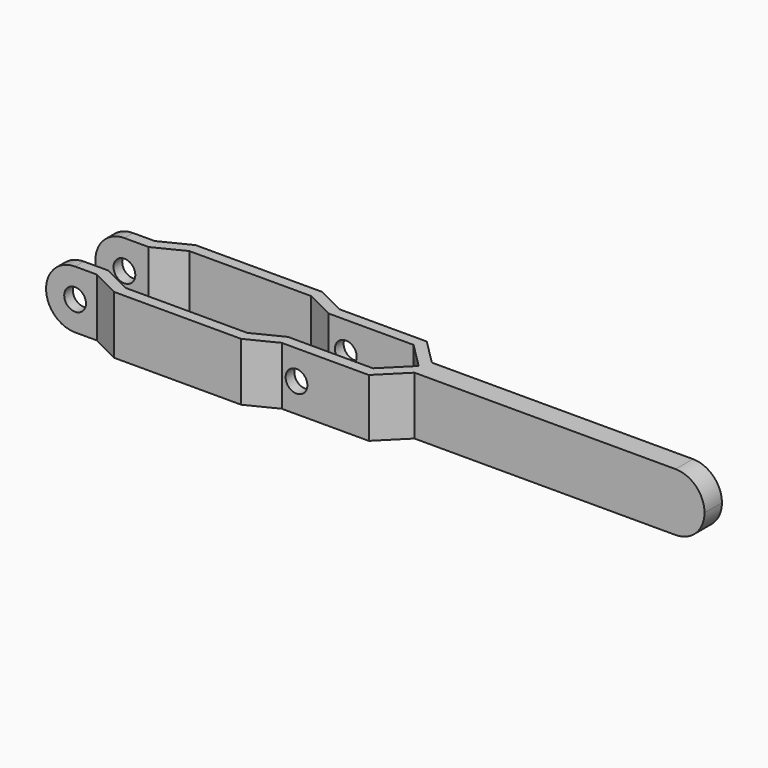
from build123d import *

# Parameters (mm, degrees)
F1_DEPTH = 16
F3_W     = 3
F3_H     = 16
F5_DEPTH = 8
F4_W     = 6
F4_H     = 16
F6_DEPTH = 8
F7_D     = 6
F8_R     = 7.99999


# Not quite as in the source:
# - a fillet or chamfer is up to 0.001 mm smaller than in the source, because OpenCascade refuses the exact size


with BuildPart() as f1:
    # F0 (on Top) → F1 (new body)
    with BuildSketch(Plane.XY):
        Polygon((-80.7573593129, 10), (-86.7573593129, 10), (-86.7573593129, 7), (-80.0491553804, 7), (-72.0491553804, 11), (-38.4655632454, 11), (-30.4655632454, 7), (-7, 7), (0, 0), (-7, -7), (-30.4655632454, -7), (-38.4655632454, -11), (-72.0491553804, -11), (-80.0491553804, -7), (-86.7573593129, -7), (-86.7573593129, -10), (-80.7573593129, -10), (-72.7573593129, -14), (-37.7573593129, -14), (-29.7573593129, -10), (-5.7573593129, -10), (1.2426406871, -3), (73.2426406871, -3), (73.2426406871, 3), (1.2426406871, 3), (-5.7573593129, 10), (-29.7573593129, 10), (-37.7573593129, 14), (-72.7573593129, 14), align=None)
    extrude(amount=F1_DEPTH)

    # F3 (on face) → F5 (join)
    with BuildSketch(Plane(origin=(-86.7573593129, 0, 0), x_dir=(0, -1, 0), z_dir=(-1, 0, 0))):
        with Locations((-8.5, 8)):
            Rectangle(F3_W, F3_H)
        with Locations((8.5, 8)):
            Rectangle(F3_W, F3_H)
    extrude(amount=F5_DEPTH)

    # F4 (on face) → F6 (join)
    with BuildSketch(Plane.YZ.offset(73.2426406871)):
        with Locations((0, 8)):
            Rectangle(F4_W, F4_H)
    extrude(amount=F6_DEPTH)

    # F7 (through all)
    with Locations(Plane.XZ.offset(10)):
        with Locations((-86.7573593129, 8), (-25.6900005043, 8)):
            Hole(F7_D / 2)

    # F8 (radius 8 in the source; OpenCascade refuses exactly that, so slightly less here)
    f8_edges = [f1.edges().sort_by_distance(p)[0] for p in [
        (-94.757359, -8.5, 16),
        (-94.757359, -8.5, 0),
        (-94.757359, 8.5, 0),
        (-94.757359, 8.5, 16),
        (81.242641, 0, 16),
        (81.242641, 0, 0),
    ]]
    fillet(f8_edges, radius=F8_R)


solid = f1.part
